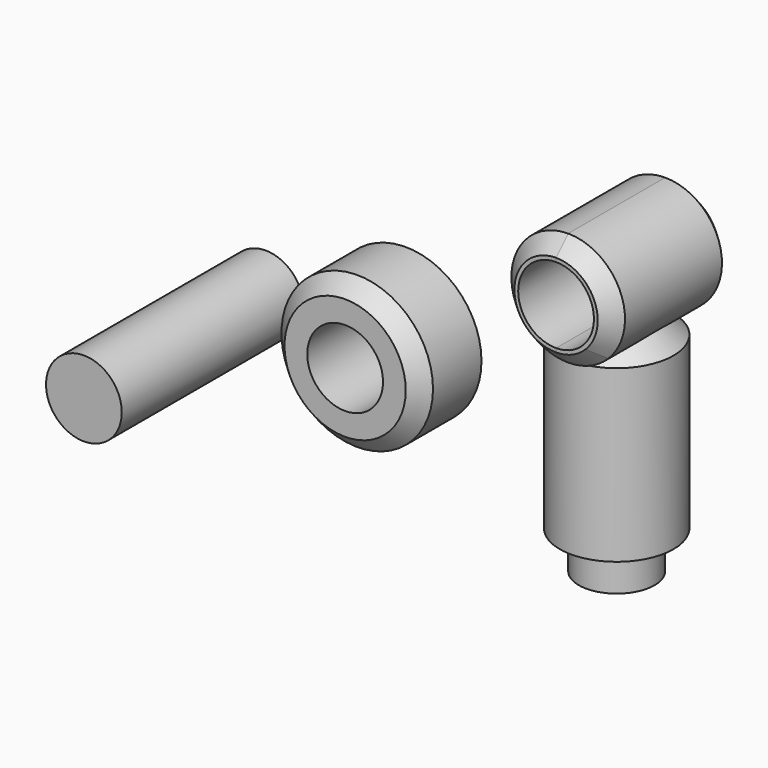
from build123d import *
from build123d import SkipClean  # not in build123d's __all__

# Parameters (mm, degrees)
F0_R     = 25.4
F0_R_2   = 12.7
F1_DEPTH = 25.4
F2_SIZE  = 5.08
F3_DEPTH = 25.4
F0_W     = 12.7
F0_H     = 12.7
F6_SIZE  = 5.08
F7_R     = 12.7
F8_DEPTH = 76.2


with BuildPart() as f1:
    # F0 (on Front) → F1 (new body)
    with BuildSketch(Plane.XZ):
        with Locations((-25.174351, 3.590025)):
            Circle(F0_R)
        with Locations((-25.174351, 3.590025)):
            Circle(F0_R_2, mode=Mode.SUBTRACT)
    extrude(amount=F1_DEPTH)

    # F2
    f2_edges = [f1.edges().sort_by_distance(p)[0] for p in [
        (-50.574351, -25.4, 3.590025),
    ]]
    chamfer(f2_edges, length=F2_SIZE)


with BuildPart() as f3:
    # F0 (on Front) → F3 (new body, symmetric)
    with BuildSketch(Plane.XZ):
        with BuildLine():
            Line((59.023077, 31.698843), (45.552693, 26.119227))
            ThreePointArc((45.552693, 26.119227), (52.842813, 27.569322), (59.023077, 31.698843))
        make_face()
        with BuildLine():
            Line((45.552693, 32.469227), (45.552693, 26.119227))
            Line((45.552693, 26.119227), (59.023077, 31.698843))
            ThreePointArc((59.023077, 31.698843), (63.152598, 52.459346), (45.552693, 64.219227))
            Line((45.552693, 64.219227), (45.552693, 57.869227))
            ThreePointArc((45.552693, 57.869227), (58.252693, 45.169227), (45.552693, 32.469227))
        make_face()
    extrude(amount=F3_DEPTH, both=True)

    # F4: F3 across face


with BuildPart() as f3_1:
    add(f3.part, clean=False)
    with SkipClean():  # cleaning this boolean's faces spoils the solid; the shape is the same uncleaned
        add(f3.part.mirror(Plane(origin=(45.552693, 0, 29.294227), x_dir=(0, -1, 0), z_dir=(-1, 0, 0))), clean=False)

    # F0 (on Front) → F5 (revolve)
    with BuildSketch(Plane.XZ):
        with BuildLine():
            ThreePointArc((59.023077, 31.698843), (52.842813, 27.569322), (45.552693, 26.119227))
            Line((45.552693, 26.119227), (45.552693, -31.030773))
            Line((45.552693, -31.030773), (58.252693, -31.030773))
            Line((58.252693, -31.030773), (64.602693, -31.030773))
            Line((64.602693, -31.030773), (64.602693, 26.119227))
            Line((64.602693, 26.119227), (59.023077, 31.698843))
        make_face()
        with Locations((51.902693, -37.380773)):
            Rectangle(F0_W, F0_H)
    with SkipClean():  # cleaning this boolean's faces spoils the solid; the shape is the same uncleaned
        revolve(axis=Axis((45.552693, 0, -2.455773), (0, 0, -1)))

    # F6
    f6_edges = [f3_1.edges().sort_by_distance(p)[0] for p in [
        (64.602693, -25.4, 45.169227),
        (26.502693, -25.4, 45.169227),
        (64.602693, 25.4, 45.169227),
        (26.502693, 25.4, 45.169227),
    ]]
    chamfer(f6_edges, length=F6_SIZE)


with BuildPart() as f8:
    # F7 (on Front) → F8 (new body)
    with BuildSketch(Plane.XZ):
        with Locations((-72.123126, 0)):
            Circle(F7_R)
    extrude(amount=F8_DEPTH)


solid = Compound([f1.part, f3_1.part, f8.part])
